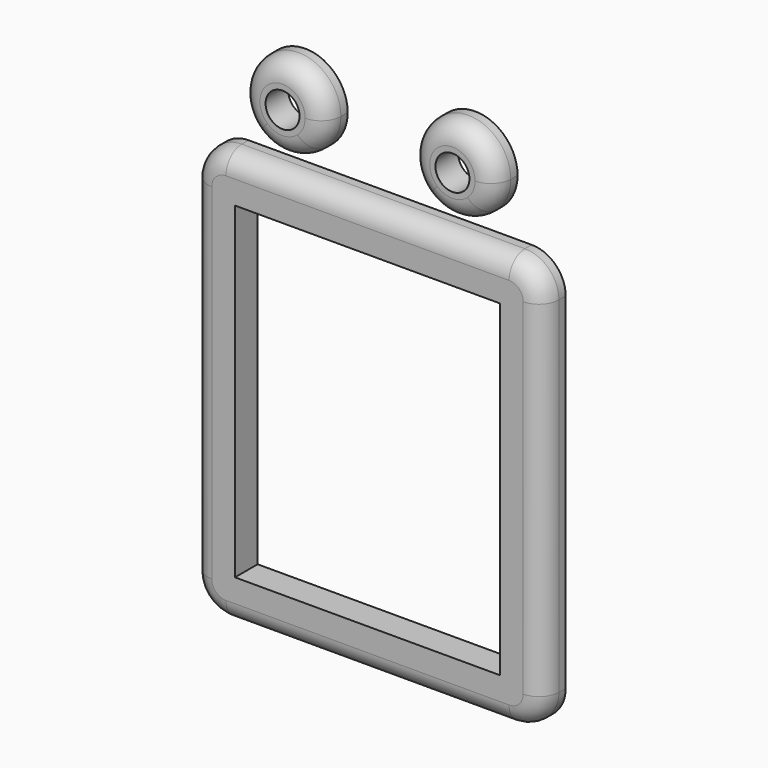
from build123d import *

# Parameters (mm, degrees)
F5_W         = 46
F5_H         = 57
F0_DEPTH     = 5
F5_R         = 3
F2_R         = 3.5
F2_2_R       = 3.5
F2_3_R       = 3.5
F3_T1_DEPTH  = 20
F3_T4_ANGLE  = 90
F3_T6_ANGLE  = 90
F3_T8_ANGLE  = 90
F3_T10_ANGLE = 90
F6_R         = 1.5
F7_W         = 46.8
F7_H         = 57.8
F7_W_2       = 46
F7_H_2       = 57
F4_DEPTH     = 5


# Not quite as in the source:
# - a fillet or chamfer that OpenCascade refuses, or shapes differently, is made with other operations: its cross-section is extruded or revolved along the edge and cut away or added
# - a feature of the source that left no trace in its solid (it failed there, or was rolled back) is left out
# - a feature names something its author has since deleted; it is built from what else it names


with BuildPart() as f0:
    # F5 (on Front) → F0 (new body)
    with BuildSketch(Plane.XZ):
        Polygon((-31, -8), (31, -8), (31, 65), (20, 65), (15.5901699437, 65), (15, 65), (10, 65), (5.5901699437, 65), (0, 65), (-5.5901699437, 65), (-10, 65), (-15, 65), (-15.5901699437, 65), (-20, 65), (-31, 65), align=None)
        with Locations((0, 28.5)):
            Rectangle(F5_W, F5_H, mode=Mode.SUBTRACT)
    extrude(amount=F0_DEPTH)

    # F2
    f2_edges = [f0.edges().sort_by_distance(p)[0] for p in [
        (31, -5, 28.5),
        (0, -5, 65),
        (-31, -5, 28.5),
        (0, -5, -8),
    ]]
    fillet(f2_edges, radius=F2_R)

    # F3: fillet of radius 6 on 4 edges, made by hand

    # F3_s2 → F3_t1 (cut)
    with BuildSketch(Plane.XZ.offset(-15)):
        with BuildLine():
            ThreePointArc((-25, -8), (-29.2426406871, -6.2426406871), (-31, -2))
            Line((-31, -2), (-31, -8))
            Line((-31, -8), (-25, -8))
        make_face()
        with BuildLine():
            ThreePointArc((-31, 59), (-29.2426406871, 63.2426406871), (-25, 65))
            Line((-25, 65), (-31, 65))
            Line((-31, 65), (-31, 59))
        make_face()
        with BuildLine():
            ThreePointArc((31, 59), (29.2426406871, 63.2426406871), (25, 65))
            Line((25, 65), (31, 65))
            Line((31, 65), (31, 59))
        make_face()
        with BuildLine():
            ThreePointArc((25, -8), (29.2426406871, -6.2426406871), (31, -2))
            Line((31, -2), (31, -8))
            Line((31, -8), (25, -8))
        make_face()
    extrude(amount=F3_T1_DEPTH, mode=Mode.SUBTRACT)

    # F3_s3 → F3_t4 (revolve, cut)
    with BuildSketch(Plane.YZ.offset(25)):
        with BuildLine():
            ThreePointArc((-5, -4.5), (-3.9748737342, -6.9748737342), (-1.5, -8))
            Line((-1.5, -8), (-5, -8))
            Line((-5, -8), (-5, -4.5))
        make_face()
    revolve(axis=Axis((25, -5, -2), (0, -1, 0)), revolution_arc=F3_T4_ANGLE, mode=Mode.SUBTRACT)

    # F3_s5 → F3_t6 (revolve, cut)
    with BuildSketch(Plane.XY.offset(59)):
        with BuildLine():
            ThreePointArc((27.5, -5), (29.9748737342, -3.9748737342), (31, -1.5))
            Line((31, -1.5), (31, -5))
            Line((31, -5), (27.5, -5))
        make_face()
    revolve(axis=Axis((25, -5, 59), (0, -1, 0)), revolution_arc=F3_T6_ANGLE, mode=Mode.SUBTRACT)

    # F3_s7 → F3_t8 (revolve, cut)
    with BuildSketch(Plane.YZ.offset(-25)):
        with BuildLine():
            ThreePointArc((-5, 61.5), (-3.9748737342, 63.9748737342), (-1.5, 65))
            Line((-1.5, 65), (-5, 65))
            Line((-5, 65), (-5, 61.5))
        make_face()
    revolve(axis=Axis((-25, -5, 59), (0, -1, 0)), revolution_arc=F3_T8_ANGLE, mode=Mode.SUBTRACT)

    # F3_s9 → F3_t10 (revolve, cut)
    with BuildSketch(Plane.XY.offset(-2)):
        with BuildLine():
            ThreePointArc((-27.5, -5), (-29.9748737342, -3.9748737342), (-31, -1.5))
            Line((-31, -1.5), (-31, -5))
            Line((-31, -5), (-27.5, -5))
        make_face()
    revolve(axis=Axis((-25, -5, -2), (0, -1, 0)), revolution_arc=F3_T10_ANGLE, mode=Mode.SUBTRACT)

    # F6
    f6_edges = [f0.edges().sort_by_distance(p)[0] for p in [
        (-23, -2.5, 57),
        (23, -2.5, 57),
        (23, -2.5, 0),
        (-23, -2.5, 0),
    ]]
    fillet(f6_edges, radius=F6_R)

    # F7 (on face) → F4 (cut, through all)
    with BuildSketch(Plane.XZ):
        with Locations((0, 28.5)):
            Rectangle(F7_W, F7_H)
        with Locations((0, 28.5)):
            Rectangle(F7_W_2, F7_H_2, mode=Mode.SUBTRACT)
        with Locations((0, 28.5)):
            Rectangle(F7_W_2, F7_H_2)
    extrude(amount=F4_DEPTH, mode=Mode.SUBTRACT)


with BuildPart() as f0b:
    # F5 (on Front) → F0, piece 2 (new body)
    with BuildSketch(Plane.XZ):
        with BuildLine():
            Line((10, 69.4098300563), (20, 69.4098300563))
            ThreePointArc((20, 69.4098300563), (21.8465319688, 71.9381378215), (22.5, 75))
            ThreePointArc((22.5, 75), (11.9381378215, 81.8465319688), (10, 69.4098300563))
        make_face()
        with Locations((15, 75)):
            Circle(F5_R, mode=Mode.SUBTRACT)
        with BuildLine():
            ThreePointArc((10, 69.4098300563), (15, 67.5), (20, 69.4098300563))
            Line((20, 69.4098300563), (10, 69.4098300563))
        make_face()
    extrude(amount=F0_DEPTH)

    # F2#2
    f2_2_edges = [f0b.edges().sort_by_distance(p)[0] for p in [
        (7.5, -5, 75),
    ]]
    fillet(f2_2_edges, radius=F2_2_R)


with BuildPart() as f0c:
    # F5 (on Front) → F0, piece 3 (new body)
    with BuildSketch(Plane.XZ):
        with BuildLine():
            Line((-10, 69.4098300563), (-20, 69.4098300563))
            ThreePointArc((-20, 69.4098300563), (-15, 67.5), (-10, 69.4098300563))
        make_face()
        with BuildLine():
            ThreePointArc((-7.5, 75), (-18.0618621785, 81.8465319688), (-20, 69.4098300563))
            Line((-20, 69.4098300563), (-10, 69.4098300563))
            ThreePointArc((-10, 69.4098300563), (-8.1534680312, 71.9381378215), (-7.5, 75))
        make_face()
        with Locations((-15, 75)):
            Circle(F5_R, mode=Mode.SUBTRACT)
    extrude(amount=F0_DEPTH)

    # F2#3
    f2_3_edges = [f0c.edges().sort_by_distance(p)[0] for p in [
        (-20, -5, 80.59017),
    ]]
    fillet(f2_3_edges, radius=F2_3_R)


solid = Compound([f0.part, f0b.part, f0c.part])
